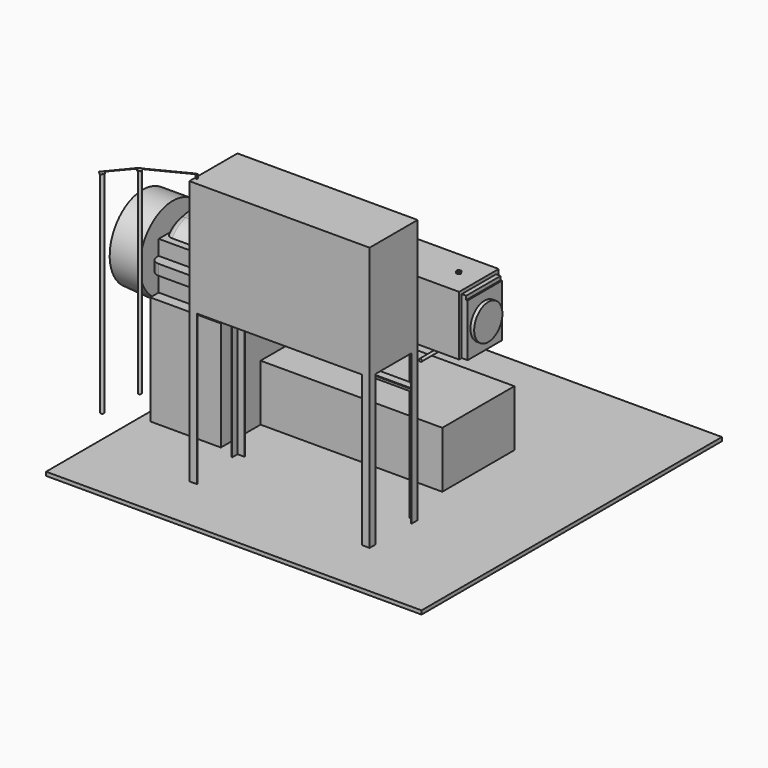
from build123d import *

# Parameters (mm, degrees)
F0_W         = 2500
F0_H         = 2500
F1_DEPTH     = 25
F3_DEPTH     = 1000
F4_W         = 1200
F4_H         = 400
F5_DEPTH     = 760
F6_W         = 1210
F6_H         = 600
F7_DEPTH     = 375
F8_W         = 470
F8_H         = 930
F9_DEPTH     = 727
F11_W        = 10.9674930573
F11_H        = 6.9268345833
F12_DEPTH    = 25
F14_DEPTH    = 1
F16_DEPTH    = 1
F17_R        = 10.4775
F18_DEPTH    = 1310
F19_R        = 10.4775
F20_DEPTH    = 1406.4
F22_DEPTH    = 470
F23_T1_DEPTH = 1149.1676659935
F24_T1_DEPTH = 1056.4932379115
F25_R        = 50
F26_R        = 55
F27_W        = 330
F27_H        = 397
F28_DEPTH    = 1210
F29_W        = 286
F29_H        = 375
F30_DEPTH    = 30
F31_W        = 286
F31_H        = 350
F32_DEPTH    = 9
F33_R        = 117.5
F34_DEPTH    = 25
F36_DEPTH    = 1200
F37_R        = 9.3155
F38_DEPTH    = 10
F39_R        = 9.3155
F40_DEPTH    = 10
F41_R        = 9.3155
F42_DEPTH    = 10
F43_R        = 9.3155
F44_DEPTH    = 13
F45_W        = 22
F45_H        = 22
F46_DEPTH    = 22
F47_W        = 22
F47_H        = 22
F48_DEPTH    = 22
F49_W        = 22
F49_H        = 22
F50_DEPTH    = 22
F51_R        = 9.3155
F52_DEPTH    = 249
F53_R        = 9.3155
F54_DEPTH    = 249
F55_R        = 9.3155
F56_DEPTH    = 93
F57_W        = 22
F57_H        = 22
F58_DEPTH    = 22
F59_R        = 9.3155
F60_DEPTH    = 249
F62_DEPTH    = 200


# Not quite as in the source:
# - a fillet or chamfer that OpenCascade refuses, or shapes differently, is made with other operations: its cross-section is extruded or revolved along the edge and cut away or added


with BuildPart() as f1:
    # F0 (on Top) → F1 (new body)
    with BuildSketch(Plane.XY):
        Rectangle(F0_W, F0_H)
    extrude(amount=F1_DEPTH)

    # F2 (on face) → F3 (join)
    with BuildSketch(Plane.XY.offset(25)):
        Polygon((-600, -520), (-595, -520), (-595, -475), (-550, -475), (-550, -470), (-600, -470), align=None)
        Polygon((595, -520), (600, -520), (600, -470), (550, -470), (550, -475), (595, -475), align=None)
        Polygon((-595, -820), (-600, -820), (-600, -870), (-550, -870), (-550, -865), (-595, -865), align=None)
        Polygon((600, -870), (600, -820), (595, -820), (595, -865), (550, -865), (550, -870), align=None)
    extrude(amount=F3_DEPTH)

    # F4 (on face) → F5 (join)
    with BuildSketch(Plane.XY.offset(1025)):
        with Locations((0, -670)):
            Rectangle(F4_W, F4_H)
    extrude(amount=F5_DEPTH)

    # F6 (on face) → F7 (join)
    with BuildSketch(Plane.XY.offset(25)):
        with Locations((-105, 160)):
            Rectangle(F6_W, F6_H)
    extrude(amount=F7_DEPTH)

    # F8 (on face) → F9 (join)
    with BuildSketch(Plane.XY.offset(25)):
        with Locations((-945, -5)):
            Rectangle(F8_W, F8_H)
    extrude(amount=F9_DEPTH)

    # F11 (on face) → F12 (join)
    with BuildSketch(Plane.XY.offset(1785)):
        with Locations((-588.548541069, -823.9167034626)):
            Rectangle(F11_W, F11_H)
    extrude(amount=F12_DEPTH)

    # F13 (on face) → F14 (join)
    with BuildSketch(Plane.XY.offset(1810)):
        Polygon((-583.0647945404, -827.3801207542), (-583.0647945404, -820.453286171), (-594.0322875977, -820.453286171), (-868.3796525002, -960.9092473984), (-853.8979996326, -989.1957171852), (-833.3796413458, -978.6910573828), (-843.3240652084, -953.7014961243), (-594.0322875977, -827.3801207542), align=None)
    extrude(amount=F14_DEPTH)

    # F15 (on face) → F16 (join)
    with BuildSketch(Plane.XY.offset(1811)):
        Polygon((-847.8612942133, -950.404587596), (-868.3796525002, -960.9092473984), (-1001.0491609573, -1121.7446327209), (-979.0826439857, -1142.681479454), (-959.1100018946, -1121.7265865298), (-979.0826439857, -1100.8077859879), (-865.6047218848, -966.3294153675), (-853.8979996326, -989.1957171852), (-833.3796413458, -978.6910573828), align=None)
    extrude(amount=F16_DEPTH)

    # F17 (on face) → F18 (join)
    with BuildSketch(Plane(origin=(0, 0, 1810), x_dir=(1, 0, 0), z_dir=(0, 0, -1))):
        with Locations((-850, 970)):
            Circle(F17_R)
    extrude(amount=F18_DEPTH)

    # F19 (on face) → F20 (join)
    with BuildSketch(Plane(origin=(0, 0, 1811), x_dir=(1, 0, 0), z_dir=(0, 0, -1))):
        with Locations((-980, 1120)):
            Circle(F19_R)
    extrude(amount=F20_DEPTH)

    # F21 (on face) → F22 (join)
    with BuildSketch(Plane(origin=(-1180, 0, 0), x_dir=(0, -1, 0), z_dir=(-1, 0, 0))):
        Polygon((-390, 675.8737691168), (400, 675.8737691168), (400, 897), (470, 897), (470, 967), (400, 967), (400, 1067), (351.8749655669, 1067), (351.8749655669, 1117), (-290, 1252), (-290, 1152), (-390, 1152), (-390, 1052), (-460, 1052), (-460, 982), (-390, 982), align=None)
    extrude(amount=-F22_DEPTH)

    # F23: fillet of radius 116.7973100446 on 1 edges, made by hand

    # F23_s2 → F23_t1 (cut)
    with BuildSketch(Plane.YZ.offset(-1519.5838329968)):
        with BuildLine():
            ThreePointArc((290, 1152), (236.7671774556, 1212.4316923823), (157.0746350758, 1224.0429597236))
            Line((157.0746350758, 1224.0429597236), (290, 1252))
            Line((290, 1252), (290, 1152))
        make_face()
    extrude(amount=F23_T1_DEPTH, mode=Mode.SUBTRACT)

    # F24: fillet of radius 190.8173067118 on 1 edges, made by hand

    # F24_s2 → F24_t1 (cut)
    with BuildSketch(Plane.YZ.offset(-1473.2466189558)):
        with BuildLine():
            ThreePointArc((-237.0876581339, 1141.142219801), (-301.3458097176, 1114.6987553793), (-351.8749655669, 1067))
            Line((-351.8749655669, 1067), (-351.8749655669, 1117))
            Line((-351.8749655669, 1117), (-237.0876581339, 1141.142219801))
        make_face()
    extrude(amount=F24_T1_DEPTH, mode=Mode.SUBTRACT)

    # F25
    f25_edges = [f1.edges().sort_by_distance(p)[0] for p in [
        (-710, -40.006512, 1182.59259),
        (-1180, -40.006512, 1182.59259),
        (-710, 236.767177, 1212.431692),
        (-710, -301.34581, 1114.698755),
        (-1180, 236.767177, 1212.431692),
    ]]
    fillet(f25_edges, radius=F25_R)

    # F26
    f26_edges = [f1.edges().sort_by_distance(p)[0] for p in [
        (-710, 460, 1017),
        (-1180, 460, 1017),
        (-1180, -470, 932),
        (-710, -470, 932),
    ]]
    fillet(f26_edges, radius=F26_R)

    # F27 (on face) → F28 (join)
    with BuildSketch(Plane.YZ.offset(-710)):
        with Locations((165, 941.5)):
            Rectangle(F27_W, F27_H)
    extrude(amount=F28_DEPTH)

    # F29 (on face) → F30 (join)
    with BuildSketch(Plane.YZ.offset(500)):
        with Locations((165, 930.5)):
            Rectangle(F29_W, F29_H)
    extrude(amount=F30_DEPTH)

    # F31 (on face) → F32 (join)
    with BuildSketch(Plane.YZ.offset(530)):
        with Locations((165, 918)):
            Rectangle(F31_W, F31_H)
    extrude(amount=F32_DEPTH)

    # F33 (on face) → F34 (join)
    with BuildSketch(Plane.YZ.offset(539)):
        with Locations((163.0614250898, 917.7260994911)):
            Circle(F33_R)
    extrude(amount=F34_DEPTH)

    # F35 (on face) → F36 (join)
    with BuildSketch(Plane.YZ.offset(600)):
        Polygon((-470, 818), (-520, 818), (-520, 813), (-475, 813), (-475, 768), (-470, 768), align=None)
    extrude(amount=-F36_DEPTH)

    # F37 (on face) → F38 (join)
    with BuildSketch(Plane.XY.offset(1140)):
        Polygon((357.4944465005, 152), (372.5055534995, 152), (380.0111069989, 165), (372.5055534995, 178), (357.4944465005, 178), (349.9888930011, 165), align=None)
        with Locations((365, 165)):
            Circle(F37_R, mode=Mode.SUBTRACT)
    extrude(amount=F38_DEPTH)

    # F39 (on face) → F40 (join)
    with BuildSketch(Plane.XY.offset(1140)):
        Polygon((28.2709041504, 152.4730100236), (34.9841436277, 165.8993181183), (26.7132394773, 178.4263080947), (11.7290958496, 177.5269899764), (5.0158563723, 164.1006818817), (13.2867605227, 151.5736919053), align=None)
        with Locations((20, 165)):
            Circle(F39_R, mode=Mode.SUBTRACT)
    extrude(amount=F40_DEPTH)

    # F41 (on face) → F42 (join)
    with BuildSketch(Plane.XY.offset(1140)):
        Polygon((-307, 127.4944465005), (-307, 142.5055534995), (-320, 150.0111069989), (-333, 142.5055534995), (-333, 127.4944465005), (-320, 119.9888930011), align=None)
        with Locations((-320, 135)):
            Circle(F41_R, mode=Mode.SUBTRACT)
    extrude(amount=F42_DEPTH)

    # F43 (on face) → F44 (join)
    with BuildSketch(Plane(origin=(0, 0, 743), x_dir=(1, 0, 0), z_dir=(0, 0, -1))):
        with Locations((319, -165)):
            Circle(F43_R)
        with Locations((-21, -165)):
            Circle(F43_R)
        with Locations((-261, -165)):
            Circle(F43_R)
    extrude(amount=F44_DEPTH)

    # F45 (on face) → F46 (join)
    with BuildSketch(Plane(origin=(0, 0, 730), x_dir=(1, 0, 0), z_dir=(0, 0, -1))):
        with Locations((319, -165)):
            Rectangle(F45_W, F45_H)
    extrude(amount=F46_DEPTH)

    # F47 (on face) → F48 (join)
    with BuildSketch(Plane(origin=(0, 0, 730), x_dir=(1, 0, 0), z_dir=(0, 0, -1))):
        with Locations((-21, -165)):
            Rectangle(F47_W, F47_H)
    extrude(amount=F48_DEPTH)

    # F49 (on face) → F50 (join)
    with BuildSketch(Plane(origin=(0, 0, 730), x_dir=(1, 0, 0), z_dir=(0, 0, -1))):
        with Locations((-261, -165)):
            Rectangle(F49_W, F49_H)
    extrude(amount=F50_DEPTH)

    # F51 (on face) → F52 (join)
    with BuildSketch(Plane.XZ.offset(-154)):
        with Locations((-21, 719)):
            Circle(F51_R)
    extrude(amount=F52_DEPTH)

    # F53 (on face) → F54 (join)
    with BuildSketch(Plane.XZ.offset(-154)):
        with Locations((319, 719)):
            Circle(F53_R)
    extrude(amount=F54_DEPTH)

    # F55 (on face) → F56 (join)
    with BuildSketch(Plane.YZ.offset(-250)):
        with Locations((165, 719)):
            Circle(F55_R)
    extrude(amount=F56_DEPTH)

    # F57 (on face) → F58 (join)
    with BuildSketch(Plane.YZ.offset(-157)):
        with Locations((165, 719)):
            Rectangle(F57_W, F57_H)
    extrude(amount=F58_DEPTH)

    # F59 (on face) → F60 (join)
    with BuildSketch(Plane.XZ.offset(-154)):
        with Locations((-146, 719)):
            Circle(F59_R)
    extrude(amount=F60_DEPTH)

    # F61 (on face) → F62 (join)
    with BuildSketch(Plane(origin=(-1180, 0, 0), x_dir=(0, -1, 0), z_dir=(-1, 0, 0))):
        with BuildLine():
            ThreePointArc((455.0323445535, 752), (531.020282561, 847.7803531833), (558.1259755323, 967))
            ThreePointArc((558.1259755323, 967), (382.1362992227, 1224.0624261465), (78.8194098066, 1152.9827405902))
            Line((78.8194098066, 1152.9827405902), (44.0595805352, 1105.6693669088))
            ThreePointArc((44.0595805352, 1105.6693669088), (92.8146737356, 766.7707470249), (433.8704965318, 736.6002414113))
            Line((433.8704965318, 736.6002414113), (455.0323445535, 752))
        make_face()
        with BuildLine():
            Line((44.0595805352, 1105.6693669088), (78.8194098066, 1152.9827405902))
            ThreePointArc((78.8194098066, 1152.9827405902), (60.1766677259, 1130.2538182054), (44.0595805352, 1105.6693669088))
        make_face()
        with BuildLine():
            ThreePointArc((433.8704965318, 736.6002414113), (444.6342358888, 744.0489017954), (455.0323445535, 752))
            Line((455.0323445535, 752), (433.8704965318, 736.6002414113))
        make_face()
        with BuildLine():
            ThreePointArc((433.8704965318, 736.6002414113), (92.8146737356, 766.7707470249), (44.0595805352, 1105.6693669088))
            Line((44.0595805352, 1105.6693669088), (-525.3029733187, 330.6810014486))
            ThreePointArc((-525.3029733187, 330.6810014486), (-404.1330620119, 336.3259139405), (-341.8596304295, 232.2296500206))
            ThreePointArc((-341.8596304295, 232.2296500206), (-354.7156292566, 178.6353574194), (-390.4856540295, 136.7052938252))
            Line((-390.4856540295, 136.7052938252), (433.8704965318, 736.6002414113))
        make_face()
        with BuildLine():
            ThreePointArc((-341.8596304295, 232.2296500206), (-404.1330620119, 336.3259139405), (-525.3029733187, 330.6810014486))
            ThreePointArc((-525.3029733187, 330.6810014486), (-557.0107092124, 164.8051053773), (-390.4856540295, 136.7052938252))
            ThreePointArc((-390.4856540295, 136.7052938252), (-354.7156292566, 178.6353574194), (-341.8596304295, 232.2296500206))
        make_face()
    extrude(amount=F62_DEPTH)


solid = f1.part
